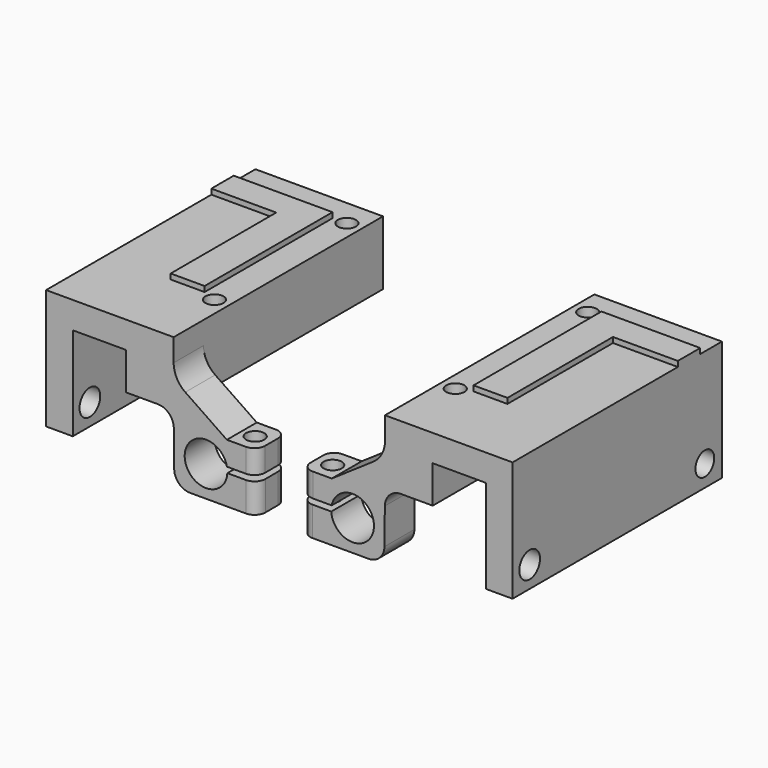
from build123d import *

# Parameters (mm, degrees)
F1_DEPTH      = 7
F2_DEPTH      = 42
F3_R          = 1.7
F3_R_2        = 11
F4_DEPTH      = 12.001
F5_R          = 4
F6_DEPTH      = 10
F7_DEPTH      = 12.001
F8_R          = 1.4
F9_DEPTH      = 10.9920075553
F8_R_2        = 1.7
F10_DEPTH     = 4.4348209087
F11_R         = 5
F12_R         = 3
F13_R         = 3
F14_R         = 2
F15_R         = 2.2
F15_R_2       = 2.4255023423
F16_DEPTH     = 6
F17_TEXT_SIZE = 41.9437823343
F18_DEPTH     = 1


# Not quite as in the source:
# - a feature names something its author has since deleted; it is built from what else it names
# - Text() gives the source's letters only with a copy of the font that has no kerning and outlines rounded to 1/6400 em; it was checked with that copy


with BuildPart() as f1:
    # F0 (on Front) → F1 (new body)
    with BuildSketch(Plane.XZ):
        Polygon((-18.6721007523, 29.8099789735), (-18.6721007523, 7.3259699669), (-13.6721007523, 7.3259699669), (-13.6721007523, 24.8099789735), (-3.7221007523, 24.8099789735), (-3.7221007523, 17.8099789735), (5.2137966118, 17.8099789735), (5.2137966118, 22.9406704692), (5.2137966118, 29.8099789735), align=None)
        Polygon((15.1801751077, 16.1394868046), (5.2137966118, 22.9406704692), (5.2137966118, 17.8099789735), (5.3440201178, 5.1484792493), (20.7686601057, 5.1484792493), (20.7686601057, 10.6682249423), (13.4360510706, 10.6682249423), (13.4360510706, 11.7046658959), (20.7396428882, 11.7046658959), (20.7396428882, 16.1394868046), align=None)
    extrude(amount=F1_DEPTH)

    # F0 (on Front) → F2 (join)
    with BuildSketch(Plane.XZ):
        Polygon((-18.6721007523, 29.8099789735), (-18.6721007523, 7.3259699669), (-13.6721007523, 7.3259699669), (-13.6721007523, 24.8099789735), (-3.7221007523, 24.8099789735), (-3.7221007523, 17.8099789735), (5.2137966118, 17.8099789735), (5.2137966118, 22.9406704692), (5.2137966118, 29.8099789735), align=None)
    extrude(amount=-F2_DEPTH)

    # F3 (on face) → F4 (cut, through all)
    with BuildSketch(Plane(origin=(0, 0, 17.8099789735), x_dir=(1, 0, 0), z_dir=(0, 0, -1))):
        with Locations((2.4537966118, -6)):
            Circle(F3_R)
        with Locations((2.4537966118, -37)):
            Circle(F3_R)
        with Locations((17.9537966118, -21.5)):
            Circle(F3_R_2)
    extrude(amount=-F4_DEPTH, mode=Mode.SUBTRACT)

    # F5 (on face) → F6 (cut)
    with BuildSketch(Plane.XZ.offset(7)):
        with Locations((11.2778992477, 10.8989789735)):
            Circle(F5_R)
    extrude(amount=-F6_DEPTH, mode=Mode.SUBTRACT)

    # F3 (on face) → F7 (cut, through all)
    with BuildSketch(Plane(origin=(0, 0, 17.8099789735), x_dir=(1, 0, 0), z_dir=(0, 0, -1))):
        with Locations((2.4537966118, -6)):
            Circle(F3_R)
        with Locations((2.4537966118, -37)):
            Circle(F3_R)
        with Locations((17.9537966118, -21.5)):
            Circle(F3_R_2)
    extrude(amount=-F7_DEPTH, mode=Mode.SUBTRACT)

    # F8 (on face) → F9 (cut, through all)
    with BuildSketch(Plane.XY.offset(16.1394868046)):
        with Locations((17.7396428882, -3.5767070949)):
            Circle(F8_R)
    extrude(amount=-F9_DEPTH, mode=Mode.SUBTRACT)

    # F8 (on face) → F10 (cut, through all)
    with BuildSketch(Plane.XY.offset(16.1394868046)):
        with Locations((17.7396428882, -3.5767070949)):
            Circle(F8_R_2)
        with Locations((17.7396428882, -3.5767070949)):
            Circle(F8_R, mode=Mode.SUBTRACT)
    extrude(amount=-F10_DEPTH, mode=Mode.SUBTRACT)

    # F11
    f11_edges = [f1.edges().sort_by_distance(p)[0] for p in [
        (5.213797, -3.5, 22.94067),
    ]]
    fillet(f11_edges, radius=F11_R)

    # F12
    f12_edges = [f1.edges().sort_by_distance(p)[0] for p in [
        (5.213797, -3.5, 17.809979),
    ]]
    fillet(f12_edges, radius=F12_R)

    # F13
    f13_edges = [f1.edges().sort_by_distance(p)[0] for p in [
        (5.34402, -3.5, 5.148479),
    ]]
    fillet(f13_edges, radius=F13_R)

    # F14
    f14_edges = [f1.edges().sort_by_distance(p)[0] for p in [
        (20.739643, -7, 13.922076),
        (20.76866, -7, 7.908352),
        (20.739643, 0, 13.922076),
        (20.76866, 0, 7.908352),
    ]]
    fillet(f14_edges, radius=F14_R)

    # F15 (on face) → F16 (cut)
    with BuildSketch(Plane(origin=(-18.6721007523, 0, 0), x_dir=(0, -1, 0), z_dir=(-1, 0, 0))):
        with Locations((-38, 11.3259699669)):
            Circle(F15_R)
        with Locations((3, 11.3259699669)):
            Circle(F15_R_2)
    extrude(amount=-F16_DEPTH, mode=Mode.SUBTRACT)

    # F17 (on face) → F18 (join)
    with BuildSketch(Plane.XY.offset(29.8099789735)):
        with Locations(Location((3.5908724648, 36.9253193088), (0, 0, 180))):
            Text('L', F17_TEXT_SIZE, font='Open Sans', font_style=FontStyle.BOLD, text_align=(TextAlign.LEFT, TextAlign.BOTTOM))
    extrude(amount=F18_DEPTH)


with BuildPart() as f19_1:
    # F19: instance of F1
    add(f1.part.mirror(Plane.YZ))


with BuildPart() as f19_1_1:
    # F20: moved
    add(f19_1.part.moved(Location((50, 0, 0))))


solid = Compound([f1.part, f19_1_1.part])
